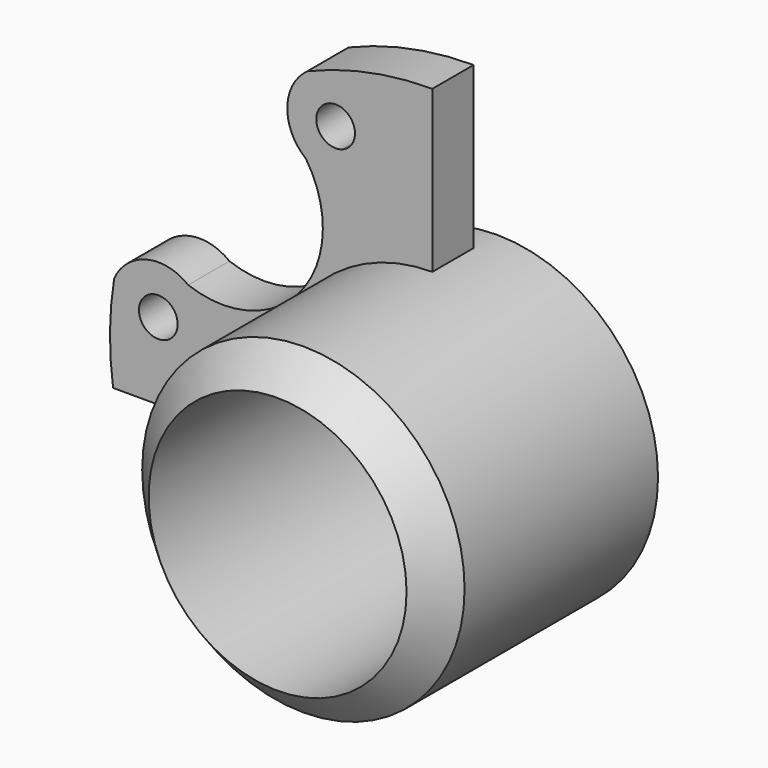
from build123d import *

# Parameters (mm, degrees)
F0_R     = 50
F0_R_2   = 40
F1_DEPTH = 85
F4_DEPTH = 16
F6_DEPTH = 18
F8_DEPTH = 17
F9_SIZE  = 9.99999


# Not quite as in the source:
# - a fillet or chamfer is up to 0.001 mm smaller than in the source, because OpenCascade refuses the exact size
# - a feature names something its author has since deleted; it is built from what else it names


with BuildPart() as f1:
    # F0 (on Front) → F1 (new body)
    with BuildSketch(Plane.XZ):
        Circle(F0_R)
        Circle(F0_R_2, mode=Mode.SUBTRACT)
    extrude(amount=F1_DEPTH)

    # F3 (on offset) → F4 (join)
    with BuildSketch(Plane.XZ.offset(9)):
        with BuildLine():
            ThreePointArc((-48.0294117647, -13.898762734), (-39.9683508335, 30.0421525802), (0, 50))
            Line((0, 50), (0, 100))
            ThreePointArc((0, 100), (-75.4648138983, 65.6129702368), (-99.0294117647, -13.898762734))
            Line((-99.0294117647, -13.898762734), (-48.0294117647, -13.898762734))
        make_face()
    extrude(amount=F4_DEPTH)

    # F5 (on offset) → F6 (cut)
    with BuildSketch(Plane.XZ.offset(9)):
        with BuildLine():
            ThreePointArc((-24, 80), (-34.9315537053, 83.4175690266), (-27.8932593505, 74.3820249346))
            ThreePointArc((-27.8932593505, 74.3820249346), (-25.0684462947, 76.5824309734), (-24, 80))
        make_face()
        with BuildLine():
            ThreePointArc((-79, 10), (-90.989717095, 10.3511255077), (-79.0410963741, 9.2989525146))
            ThreePointArc((-79.0410963741, 9.2989525146), (-79.010282905, 9.6488744923), (-79, 10))
        make_face()
    extrude(amount=F6_DEPTH, mode=Mode.SUBTRACT)

    # F7 (on face) → F8 (cut)
    with BuildSketch(Plane.XZ.offset(25)):
        with BuildLine():
            ThreePointArc((-75.732676721, 21.7947750823), (-40.5874083787, 31.7115351547), (-39.267323279, 68.2052249177))
            ThreePointArc((-39.267323279, 68.2052249177), (-44.9963531804, 80.3307435394), (-38.7382990756, 92.1918878466))
            ThreePointArc((-38.7382990756, 92.1918878466), (-78.5370863203, 61.9025530355), (-98.6907067749, 16.1289924134))
            ThreePointArc((-98.6907067749, 16.1289924134), (-88.5940024625, 24.5630747543), (-75.732676721, 21.7947750823))
        make_face()
    extrude(amount=-F8_DEPTH, mode=Mode.SUBTRACT)

    # F9 (size 10 in the source; OpenCascade refuses exactly that, so slightly less here)
    f9_edges = [f1.edges().sort_by_distance(p)[0] for p in [
        (-50, -85, 0),
    ]]
    chamfer(f9_edges, length=F9_SIZE)


solid = f1.part
